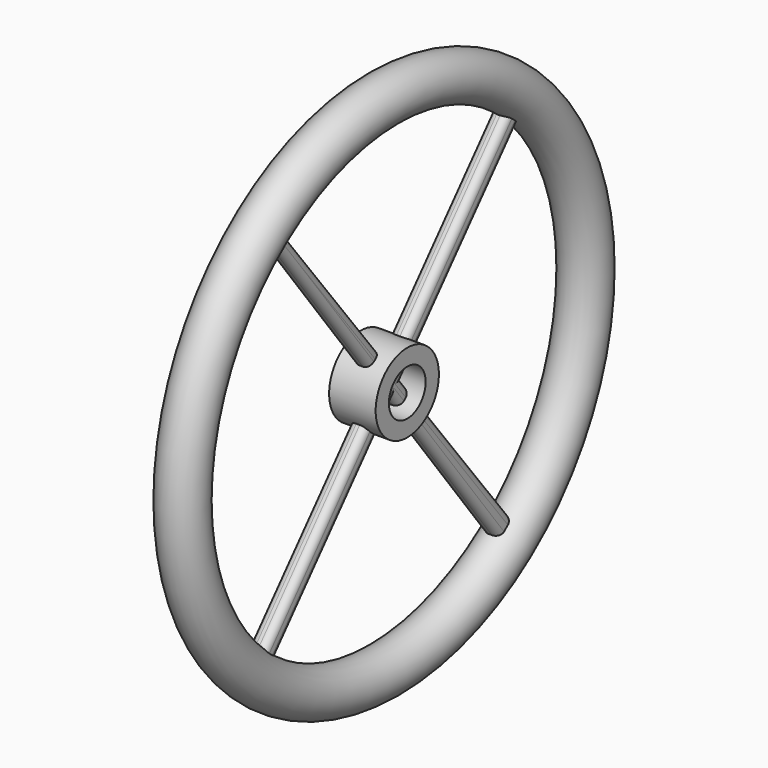
from build123d import *

# Parameters (mm, degrees)
F0_R          = 12.9236149617
F2_R          = 22.4555879502
F2_R_2        = 13.0373561963
F3_DEPTH      = 13.208
F5_DEPTH      = 4.826
F6_T1_DEPTH   = 9.652
F6_T3_DEPTH   = 28.9681227125
F6_T8_DEPTH   = 155.9510873217
F6_T13_DEPTH  = 155.9510873217
F6_T18_DEPTH  = 155.8155104326
F6_T23_DEPTH  = 155.8155104326
F6_T28_DEPTH  = 159.2863039853
F6_T33_DEPTH  = 159.2863039853
F6_T38_DEPTH  = 159.2863039853
F6_T43_DEPTH  = 159.2863039853
F6_T48_DEPTH  = 160.7409827394
F6_T53_DEPTH  = 160.7409827394
F6_T58_DEPTH  = 160.7409827394
F6_T63_DEPTH  = 160.7409827394
F6_T68_DEPTH  = 154.8184838298
F6_T73_DEPTH  = 154.8184838298
F6_T78_DEPTH  = 152.8193500484
F6_T83_DEPTH  = 152.8193500484
F6_T89_DEPTH  = 155.8155104326
F6_T93_DEPTH  = 155.9510873217
F6_T100_DEPTH = 155.8155104326
F6_T104_DEPTH = 155.9510873217
F6_T111_DEPTH = 154.8184838298
F6_T115_DEPTH = 159.2863039853
F6_T123_DEPTH = 154.8184838298
F6_T127_DEPTH = 159.2863039853
F6_T135_DEPTH = 151.0829213832
F6_T140_DEPTH = 143.1612886921
F6_T147_DEPTH = 151.0829213832
F6_T152_DEPTH = 143.1612886921
F6_T155_DEPTH = 144.3300677498
F6_T157_DEPTH = 146.2849391686
F6_T160_ANGLE = 78.1252953606
F6_T162_ANGLE = 78.1252953606


# Not quite as in the source:
# - a fillet or chamfer that OpenCascade refuses, or shapes differently, is made with other operations: its cross-section is extruded or revolved along the edge and cut away or added


with BuildPart() as f1:
    # F0 (on Front) → F1 (revolve)
    with BuildSketch(Plane.XZ):
        with Locations((0, 143.0430114269)):
            Circle(F0_R)
    revolve(axis=Axis((2.834841609, 0, 0), (1, 0, 0)))


with BuildPart() as f3:
    # F2 (on Right) → F3 (new body, symmetric)
    with BuildSketch(Plane.YZ):
        Circle(F2_R)
        Circle(F2_R_2, mode=Mode.SUBTRACT)
    extrude(amount=F3_DEPTH, both=True)


with BuildPart() as f5:
    # F4 (on Right) → F5 (new body, symmetric)
    with BuildSketch(Plane.YZ):
        Polygon((-83.4880173206, 116.8475523591), (-88.8398140669, 111.8525341153), (-5.84884804, 1.8371956864), (0.3858627438, 8.9852058397), align=None)
        Polygon((0.3858627438, 8.9852058397), (-5.84884804, 1.8371956864), (0.591610338, -6.7004710261), (6.9312324452, 0.5678185163), align=None)
        Polygon((0.591610338, -6.7004710261), (-5.84884804, 1.8371956864), (-100.2569794655, -106.4004283804), (-92.3700059439, -113.2796853781), align=None)
        Polygon((6.9312324452, 0.5678185163), (0.591610338, -6.7004710261), (80.9905081987, -113.2796853781), (90.1098596531, -106.4004283804), align=None)
        Polygon((90.1098596531, 111.8525341153), (0.3858627438, 8.9852058397), (6.9312324452, 0.5678185163), (98.9366569506, 106.0507721491), align=None)
    extrude(amount=F5_DEPTH, both=True)

    # F6: fillet of radius 3.8632245425 on 18 edges, made by hand

    # F6_s2 → F6_t1 (join)
    with BuildSketch(Plane.YZ.offset(-4.826)):
        with BuildLine():
            ThreePointArc((-7.9097995988, -0.5256569268), (-6.9603727243, 1.8766572944), (-7.7370489668, 4.3402520301))
            Line((-7.7370489668, 4.3402520301), (-5.84884804, 1.8371956864))
            Line((-5.84884804, 1.8371956864), (-7.9097995988, -0.5256569268))
        make_face()
    extrude(amount=F6_T1_DEPTH)

    # F6_s4 → F6_t3 (cut)
    with BuildSketch(Plane.YZ.offset(-14.4840613563)):
        with BuildLine():
            ThreePointArc((-97.7175985005, -103.489063034), (-98.6604928334, -106.2914766776), (-97.3456141191, -108.9398093454))
            Line((-97.3456141191, -108.9398093454), (-100.2569794655, -106.4004283804))
            Line((-100.2569794655, -106.4004283804), (-97.7175985005, -103.489063034))
        make_face()
    extrude(amount=F6_T3_DEPTH, mode=Mode.SUBTRACT)


with BuildPart() as f6_tool6:
    # F6_s7 → F6_t8 (new body)
    with BuildSketch(Plane(origin=(0, 1.7199108153, -2.2118163152), x_dir=(1, 0, 0), z_dir=(0, -0.6138537109, 0.7894198006))):
        with BuildLine():
            ThreePointArc((4.826, 1.9569850957), (3.6944877287, 4.688697367), (0.9627754575, 5.8202096382))
            Line((0.9627754575, 5.8202096382), (4.826, 5.8202096382))
            Line((4.826, 5.8202096382), (4.826, 1.9569850957))
        make_face()
    extrude(amount=F6_T8_DEPTH)

    split(bisect_by=Plane(origin=(0, -4.2318074253, 3.6911105082), x_dir=(1, 0, 0), z_dir=(0, -0.7536101809, 0.6573216071)), keep=Keep.TOP)


with BuildPart() as f5_1:
    add(f5.part)

    # F6_t5: cut F6_tool6
    add(f6_tool6.part, mode=Mode.SUBTRACT)


with BuildPart() as f6_tool11:
    # F6_s12 → F6_t13 (new body)
    with BuildSketch(Plane(origin=(0, 1.7199108153, -2.2118163152), x_dir=(1, 0, 0), z_dir=(0, -0.6138537109, 0.7894198006))):
        with BuildLine():
            ThreePointArc((-4.826, 1.9569850957), (-3.6944877287, 4.688697367), (-0.9627754575, 5.8202096382))
            Line((-0.9627754575, 5.8202096382), (-4.826, 5.8202096382))
            Line((-4.826, 5.8202096382), (-4.826, 1.9569850957))
        make_face()
    extrude(amount=F6_T13_DEPTH)

    split(bisect_by=Plane(origin=(0, -4.2318074253, 3.6911105082), x_dir=(1, 0, 0), z_dir=(0, -0.7536101809, 0.6573216071)), keep=Keep.TOP)


with BuildPart() as f5_2:
    add(f5_1.part)

    # F6_t10: cut F6_tool11
    add(f6_tool11.part, mode=Mode.SUBTRACT)


with BuildPart() as f6_tool16:
    # F6_s17 → F6_t18 (new body)
    with BuildSketch(Plane(origin=(0, 100.690119491, 115.4398369732), x_dir=(1, 0, 0), z_dir=(0, -0.6573216071, -0.7536101809))):
        with BuildLine():
            ThreePointArc((4.826, 1.7521553083), (3.6944877287, 4.4838675795), (0.9627754575, 5.6153798508))
            Line((0.9627754575, 5.6153798508), (4.826, 5.6153798508))
            Line((4.826, 5.6153798508), (4.826, 1.7521553083))
        make_face()
    extrude(amount=F6_T18_DEPTH)

    split(bisect_by=Plane(origin=(0, 4.5945887322, 3.5727572847), x_dir=(1, 0, 0), z_dir=(0, 0.7894198006, 0.6138537109)), keep=Keep.TOP)


with BuildPart() as f5_3:
    add(f5_2.part)

    # F6_t15: cut F6_tool16
    add(f6_tool16.part, mode=Mode.SUBTRACT)


with BuildPart() as f6_tool21:
    # F6_s22 → F6_t23 (new body)
    with BuildSketch(Plane(origin=(0, 100.690119491, 115.4398369732), x_dir=(1, 0, 0), z_dir=(0, -0.6573216071, -0.7536101809))):
        with BuildLine():
            ThreePointArc((-4.826, 1.7521553083), (-3.6944877287, 4.4838675795), (-0.9627754575, 5.6153798508))
            Line((-0.9627754575, 5.6153798508), (-4.826, 5.6153798508))
            Line((-4.826, 5.6153798508), (-4.826, 1.7521553083))
        make_face()
    extrude(amount=F6_T23_DEPTH)

    split(bisect_by=Plane(origin=(0, 4.5945887322, 3.5727572847), x_dir=(1, 0, 0), z_dir=(0, 0.7894198006, 0.6138537109)), keep=Keep.TOP)


with BuildPart() as f5_4:
    add(f5_3.part)

    # F6_t20: cut F6_tool21
    add(f6_tool21.part, mode=Mode.SUBTRACT)


with BuildPart() as f6_tool26:
    # F6_s27 → F6_t28 (new body)
    with BuildSketch(Plane(origin=(0, -3.0723860636, -3.5224483603), x_dir=(1, 0, 0), z_dir=(0, 0.6573216071, 0.7536101809))):
        with BuildLine():
            ThreePointArc((4.826, 0.9869834148), (3.6944877287, 3.7186956861), (0.9627754575, 4.8502079574))
            Line((0.9627754575, 4.8502079574), (4.826, 4.8502079574))
            Line((4.826, 4.8502079574), (4.826, 0.9869834148))
        make_face()
    extrude(amount=F6_T28_DEPTH)

    split(bisect_by=Plane(origin=(0, -2.8443496873, -2.1456583385), x_dir=(1, 0, 0), z_dir=(0, -0.7983268755, -0.6022243766)), keep=Keep.TOP)


with BuildPart() as f5_5:
    add(f5_4.part)

    # F6_t25: cut F6_tool26
    add(f6_tool26.part, mode=Mode.SUBTRACT)


with BuildPart() as f6_tool31:
    # F6_s32 → F6_t33 (new body)
    with BuildSketch(Plane(origin=(0, -3.0723860636, -3.5224483603), x_dir=(1, 0, 0), z_dir=(0, 0.6573216071, 0.7536101809))):
        with BuildLine():
            ThreePointArc((4.826, 0.9869834148), (3.6944877287, 3.7186956861), (0.9627754575, 4.8502079574))
            Line((0.9627754575, 4.8502079574), (4.826, 4.8502079574))
            Line((4.826, 4.8502079574), (4.826, 0.9869834148))
        make_face()
    extrude(amount=F6_T33_DEPTH)

    split(bisect_by=Plane(origin=(0, 4.5945887322, 3.5727572847), x_dir=(1, 0, 0), z_dir=(0, 0.7894198006, 0.6138537109)), keep=Keep.TOP)


with BuildPart() as f5_6:
    add(f5_5.part)

    # F6_t30: cut F6_tool31
    add(f6_tool31.part, mode=Mode.SUBTRACT)


with BuildPart() as f6_tool36:
    # F6_s37 → F6_t38 (new body)
    with BuildSketch(Plane(origin=(0, -3.0723860636, -3.5224483603), x_dir=(1, 0, 0), z_dir=(0, 0.6573216071, 0.7536101809))):
        with BuildLine():
            ThreePointArc((-4.826, 0.9869834148), (-3.6944877287, 3.7186956861), (-0.9627754575, 4.8502079574))
            Line((-0.9627754575, 4.8502079574), (-4.826, 4.8502079574))
            Line((-4.826, 4.8502079574), (-4.826, 0.9869834148))
        make_face()
    extrude(amount=F6_T38_DEPTH)

    split(bisect_by=Plane(origin=(0, -2.8443496873, -2.1456583385), x_dir=(1, 0, 0), z_dir=(0, -0.7983268755, -0.6022243766)), keep=Keep.TOP)


with BuildPart() as f5_7:
    add(f5_6.part)

    # F6_t35: cut F6_tool36
    add(f6_tool36.part, mode=Mode.SUBTRACT)


with BuildPart() as f6_tool41:
    # F6_s42 → F6_t43 (new body)
    with BuildSketch(Plane(origin=(0, -3.0723860636, -3.5224483603), x_dir=(1, 0, 0), z_dir=(0, 0.6573216071, 0.7536101809))):
        with BuildLine():
            ThreePointArc((-4.826, 0.9869834148), (-3.6944877287, 3.7186956861), (-0.9627754575, 4.8502079574))
            Line((-0.9627754575, 4.8502079574), (-4.826, 4.8502079574))
            Line((-4.826, 4.8502079574), (-4.826, 0.9869834148))
        make_face()
    extrude(amount=F6_T43_DEPTH)

    split(bisect_by=Plane(origin=(0, 4.5945887322, 3.5727572847), x_dir=(1, 0, 0), z_dir=(0, 0.7894198006, 0.6138537109)), keep=Keep.TOP)


with BuildPart() as f5_8:
    add(f5_7.part)

    # F6_t40: cut F6_tool41
    add(f6_tool41.part, mode=Mode.SUBTRACT)


with BuildPart() as f6_tool46:
    # F6_s47 → F6_t48 (new body)
    with BuildSketch(Plane(origin=(0, -102.3736244527, -117.3699522547), x_dir=(1, 0, 0), z_dir=(0, 0.6573216071, 0.7536101809))):
        with BuildLine():
            ThreePointArc((-4.826, 0.9869834148), (-3.6944877287, 3.7186956861), (-0.9627754575, 4.8502079574))
            Line((-0.9627754575, 4.8502079574), (-4.826, 4.8502079574))
            Line((-4.826, 4.8502079574), (-4.826, 0.9869834148))
        make_face()
    extrude(amount=F6_T48_DEPTH)

    split(bisect_by=Plane(origin=(0, -2.8443496873, -2.1456583385), x_dir=(1, 0, 0), z_dir=(0, -0.7983268755, -0.6022243766)), keep=Keep.TOP)


with BuildPart() as f5_9:
    add(f5_8.part)

    # F6_t45: cut F6_tool46
    add(f6_tool46.part, mode=Mode.SUBTRACT)


with BuildPart() as f6_tool51:
    # F6_s52 → F6_t53 (new body)
    with BuildSketch(Plane(origin=(0, -102.3736244527, -117.3699522547), x_dir=(1, 0, 0), z_dir=(0, 0.6573216071, 0.7536101809))):
        with BuildLine():
            ThreePointArc((-4.826, 0.9869834148), (-3.6944877287, 3.7186956861), (-0.9627754575, 4.8502079574))
            Line((-0.9627754575, 4.8502079574), (-4.826, 4.8502079574))
            Line((-4.826, 4.8502079574), (-4.826, 0.9869834148))
        make_face()
    extrude(amount=F6_T53_DEPTH)

    split(bisect_by=Plane(origin=(0, 4.5945887322, 3.5727572847), x_dir=(1, 0, 0), z_dir=(0, 0.7894198006, 0.6138537109)), keep=Keep.TOP)


with BuildPart() as f5_10:
    add(f5_9.part)

    # F6_t50: cut F6_tool51
    add(f6_tool51.part, mode=Mode.SUBTRACT)


with BuildPart() as f6_tool56:
    # F6_s57 → F6_t58 (new body)
    with BuildSketch(Plane(origin=(0, -102.3736244527, -117.3699522547), x_dir=(1, 0, 0), z_dir=(0, 0.6573216071, 0.7536101809))):
        with BuildLine():
            ThreePointArc((4.826, 0.9869834148), (3.6944877287, 3.7186956861), (0.9627754575, 4.8502079574))
            Line((0.9627754575, 4.8502079574), (4.826, 4.8502079574))
            Line((4.826, 4.8502079574), (4.826, 0.9869834148))
        make_face()
    extrude(amount=F6_T58_DEPTH)

    split(bisect_by=Plane(origin=(0, -2.8443496873, -2.1456583385), x_dir=(1, 0, 0), z_dir=(0, -0.7983268755, -0.6022243766)), keep=Keep.TOP)


with BuildPart() as f5_11:
    add(f5_10.part)

    # F6_t55: cut F6_tool56
    add(f6_tool56.part, mode=Mode.SUBTRACT)


with BuildPart() as f6_tool61:
    # F6_s62 → F6_t63 (new body)
    with BuildSketch(Plane(origin=(0, -102.3736244527, -117.3699522547), x_dir=(1, 0, 0), z_dir=(0, 0.6573216071, 0.7536101809))):
        with BuildLine():
            ThreePointArc((4.826, 0.9869834148), (3.6944877287, 3.7186956861), (0.9627754575, 4.8502079574))
            Line((0.9627754575, 4.8502079574), (4.826, 4.8502079574))
            Line((4.826, 4.8502079574), (4.826, 0.9869834148))
        make_face()
    extrude(amount=F6_T63_DEPTH)

    split(bisect_by=Plane(origin=(0, 4.5945887322, 3.5727572847), x_dir=(1, 0, 0), z_dir=(0, 0.7894198006, 0.6138537109)), keep=Keep.TOP)


with BuildPart() as f5_12:
    add(f5_11.part)

    # F6_t60: cut F6_tool61
    add(f6_tool61.part, mode=Mode.SUBTRACT)


with BuildPart() as f6_tool66:
    # F6_s67 → F6_t68 (new body)
    with BuildSketch(Plane(origin=(0, 91.4439077246, -117.5974505353), x_dir=(1, 0, 0), z_dir=(0, -0.6138537109, 0.7894198006))):
        with BuildLine():
            ThreePointArc((-4.826, 1.9569850957), (-3.6944877287, 4.688697367), (-0.9627754575, 5.8202096382))
            Line((-0.9627754575, 5.8202096382), (-4.826, 5.8202096382))
            Line((-4.826, 5.8202096382), (-4.826, 1.9569850957))
        make_face()
    extrude(amount=F6_T68_DEPTH)

    split(bisect_by=Plane(origin=(0, 3.6551660963, -3.1881464895), x_dir=(1, 0, 0), z_dir=(0, 0.7536101809, -0.6573216071)), keep=Keep.TOP)


with BuildPart() as f5_13:
    add(f5_12.part)

    # F6_t65: cut F6_tool66
    add(f6_tool66.part, mode=Mode.SUBTRACT)


with BuildPart() as f6_tool71:
    # F6_s72 → F6_t73 (new body)
    with BuildSketch(Plane(origin=(0, 91.4439077246, -117.5974505353), x_dir=(1, 0, 0), z_dir=(0, -0.6138537109, 0.7894198006))):
        with BuildLine():
            ThreePointArc((4.826, 1.9569850957), (3.6944877287, 4.688697367), (0.9627754575, 5.8202096382))
            Line((0.9627754575, 5.8202096382), (4.826, 5.8202096382))
            Line((4.826, 5.8202096382), (4.826, 1.9569850957))
        make_face()
    extrude(amount=F6_T73_DEPTH)

    split(bisect_by=Plane(origin=(0, 3.6551660963, -3.1881464895), x_dir=(1, 0, 0), z_dir=(0, 0.7536101809, -0.6573216071)), keep=Keep.TOP)


with BuildPart() as f5_14:
    add(f5_13.part)

    # F6_t70: cut F6_tool71
    add(f6_tool71.part, mode=Mode.SUBTRACT)


with BuildPart() as f6_tool76:
    # F6_s77 → F6_t78 (new body)
    with BuildSketch(Plane(origin=(0, -2.3803599544, 3.1554772586), x_dir=(1, 0, 0), z_dir=(0, 0.6022243766, -0.7983268755))):
        with BuildLine():
            ThreePointArc((-4.826, -0.3003359883), (-3.6944877287, 2.4313762829), (-0.9627754575, 3.5628885542))
            Line((-0.9627754575, 3.5628885542), (-4.826, 3.5628885542))
            Line((-4.826, 3.5628885542), (-4.826, -0.3003359883))
        make_face()
    extrude(amount=F6_T78_DEPTH)

    split(bisect_by=Plane(origin=(0, 3.6551660963, -3.1881464895), x_dir=(1, 0, 0), z_dir=(0, 0.7536101809, -0.6573216071)), keep=Keep.TOP)


with BuildPart() as f5_15:
    add(f5_14.part)

    # F6_t75: cut F6_tool76
    add(f6_tool76.part, mode=Mode.SUBTRACT)


with BuildPart() as f6_tool81:
    # F6_s82 → F6_t83 (new body)
    with BuildSketch(Plane(origin=(0, -2.3803599544, 3.1554772586), x_dir=(1, 0, 0), z_dir=(0, 0.6022243766, -0.7983268755))):
        with BuildLine():
            ThreePointArc((4.826, -0.3003359883), (3.6944877287, 2.4313762829), (0.9627754575, 3.5628885542))
            Line((0.9627754575, 3.5628885542), (4.826, 3.5628885542))
            Line((4.826, 3.5628885542), (4.826, -0.3003359883))
        make_face()
    extrude(amount=F6_T83_DEPTH)

    split(bisect_by=Plane(origin=(0, 3.6551660963, -3.1881464895), x_dir=(1, 0, 0), z_dir=(0, 0.7536101809, -0.6573216071)), keep=Keep.TOP)


with BuildPart() as f5_16:
    add(f5_15.part)

    # F6_t80: cut F6_tool81
    add(f6_tool81.part, mode=Mode.SUBTRACT)


with BuildPart() as f6_tool87:
    # F6_s88 → F6_t89 (new body)
    with BuildSketch(Plane(origin=(0, 100.690119491, 115.4398369732), x_dir=(1, 0, 0), z_dir=(0, -0.6573216071, -0.7536101809))):
        with BuildLine():
            ThreePointArc((4.826, 1.7521553083), (3.6944877287, 4.4838675795), (0.9627754575, 5.6153798508))
            Line((0.9627754575, 5.6153798508), (4.826, 5.6153798508))
            Line((4.826, 5.6153798508), (4.826, 1.7521553083))
        make_face()
    extrude(amount=F6_T89_DEPTH)

    split(bisect_by=Plane(origin=(0, 4.5945887322, 3.5727572847), x_dir=(1, 0, 0), z_dir=(0, -0.7894198006, -0.6138537109)), keep=Keep.TOP)


with BuildPart() as f6_tool91:
    # F6_s92 → F6_t93 (new body)
    with BuildSketch(Plane(origin=(0, 1.7199108153, -2.2118163152), x_dir=(1, 0, 0), z_dir=(0, -0.6138537109, 0.7894198006))):
        with BuildLine():
            ThreePointArc((4.826, 1.9569850957), (3.6944877287, 4.688697367), (0.9627754575, 5.8202096382))
            Line((0.9627754575, 5.8202096382), (4.826, 5.8202096382))
            Line((4.826, 5.8202096382), (4.826, 1.9569850957))
        make_face()
    extrude(amount=F6_T93_DEPTH)

    split(bisect_by=Plane(origin=(0, -4.2318074253, 3.6911105082), x_dir=(1, 0, 0), z_dir=(0, 0.7536101809, -0.6573216071)), keep=Keep.TOP)


with BuildPart() as f6_tool87_1:
    add(f6_tool87.part)

    # F6_t95: intersect F6_tool91
    add(f6_tool91.part, mode=Mode.INTERSECT)


with BuildPart() as f5_17:
    add(f5_16.part)

    # F6_t85: cut F6_tool87
    add(f6_tool87_1.part, mode=Mode.SUBTRACT)


with BuildPart() as f6_tool98:
    # F6_s99 → F6_t100 (new body)
    with BuildSketch(Plane(origin=(0, 100.690119491, 115.4398369732), x_dir=(1, 0, 0), z_dir=(0, -0.6573216071, -0.7536101809))):
        with BuildLine():
            ThreePointArc((-4.826, 1.7521553083), (-3.6944877287, 4.4838675795), (-0.9627754575, 5.6153798508))
            Line((-0.9627754575, 5.6153798508), (-4.826, 5.6153798508))
            Line((-4.826, 5.6153798508), (-4.826, 1.7521553083))
        make_face()
    extrude(amount=F6_T100_DEPTH)

    split(bisect_by=Plane(origin=(0, 4.5945887322, 3.5727572847), x_dir=(1, 0, 0), z_dir=(0, -0.7894198006, -0.6138537109)), keep=Keep.TOP)


with BuildPart() as f6_tool102:
    # F6_s103 → F6_t104 (new body)
    with BuildSketch(Plane(origin=(0, 1.7199108153, -2.2118163152), x_dir=(1, 0, 0), z_dir=(0, -0.6138537109, 0.7894198006))):
        with BuildLine():
            ThreePointArc((-4.826, 1.9569850957), (-3.6944877287, 4.688697367), (-0.9627754575, 5.8202096382))
            Line((-0.9627754575, 5.8202096382), (-4.826, 5.8202096382))
            Line((-4.826, 5.8202096382), (-4.826, 1.9569850957))
        make_face()
    extrude(amount=F6_T104_DEPTH)

    split(bisect_by=Plane(origin=(0, -4.2318074253, 3.6911105082), x_dir=(1, 0, 0), z_dir=(0, 0.7536101809, -0.6573216071)), keep=Keep.TOP)


with BuildPart() as f6_tool98_1:
    add(f6_tool98.part)

    # F6_t106: intersect F6_tool102
    add(f6_tool102.part, mode=Mode.INTERSECT)


with BuildPart() as f5_18:
    add(f5_17.part)

    # F6_t96: cut F6_tool98
    add(f6_tool98_1.part, mode=Mode.SUBTRACT)


with BuildPart() as f6_tool109:
    # F6_s110 → F6_t111 (new body)
    with BuildSketch(Plane(origin=(0, 91.4439077246, -117.5974505353), x_dir=(1, 0, 0), z_dir=(0, -0.6138537109, 0.7894198006))):
        with BuildLine():
            ThreePointArc((4.826, 1.9569850957), (3.6944877287, 4.688697367), (0.9627754575, 5.8202096382))
            Line((0.9627754575, 5.8202096382), (4.826, 5.8202096382))
            Line((4.826, 5.8202096382), (4.826, 1.9569850957))
        make_face()
    extrude(amount=F6_T111_DEPTH)

    split(bisect_by=Plane(origin=(0, 3.6551660963, -3.1881464895), x_dir=(1, 0, 0), z_dir=(0, -0.7536101809, 0.6573216071)), keep=Keep.TOP)


with BuildPart() as f6_tool113:
    # F6_s114 → F6_t115 (new body)
    with BuildSketch(Plane(origin=(0, -3.0723860636, -3.5224483603), x_dir=(1, 0, 0), z_dir=(0, 0.6573216071, 0.7536101809))):
        with BuildLine():
            ThreePointArc((4.826, 0.9869834148), (3.6944877287, 3.7186956861), (0.9627754575, 4.8502079574))
            Line((0.9627754575, 4.8502079574), (4.826, 4.8502079574))
            Line((4.826, 4.8502079574), (4.826, 0.9869834148))
        make_face()
    extrude(amount=F6_T115_DEPTH)

    split(bisect_by=Plane(origin=(0, -2.8443496873, -2.1456583385), x_dir=(1, 0, 0), z_dir=(0, 0.7983268755, 0.6022243766)), keep=Keep.TOP)

    split(bisect_by=Plane(origin=(0, 4.5945887322, 3.5727572847), x_dir=(1, 0, 0), z_dir=(0, -0.7894198006, -0.6138537109)), keep=Keep.TOP)


with BuildPart() as f6_tool109_1:
    add(f6_tool109.part)

    # F6_t118: intersect F6_tool113
    add(f6_tool113.part, mode=Mode.INTERSECT)


with BuildPart() as f5_19:
    add(f5_18.part)

    # F6_t107: cut F6_tool109
    add(f6_tool109_1.part, mode=Mode.SUBTRACT)


with BuildPart() as f6_tool121:
    # F6_s122 → F6_t123 (new body)
    with BuildSketch(Plane(origin=(0, 91.4439077246, -117.5974505353), x_dir=(1, 0, 0), z_dir=(0, -0.6138537109, 0.7894198006))):
        with BuildLine():
            ThreePointArc((-4.826, 1.9569850957), (-3.6944877287, 4.688697367), (-0.9627754575, 5.8202096382))
            Line((-0.9627754575, 5.8202096382), (-4.826, 5.8202096382))
            Line((-4.826, 5.8202096382), (-4.826, 1.9569850957))
        make_face()
    extrude(amount=F6_T123_DEPTH)

    split(bisect_by=Plane(origin=(0, 3.6551660963, -3.1881464895), x_dir=(1, 0, 0), z_dir=(0, -0.7536101809, 0.6573216071)), keep=Keep.TOP)


with BuildPart() as f6_tool125:
    # F6_s126 → F6_t127 (new body)
    with BuildSketch(Plane(origin=(0, -3.0723860636, -3.5224483603), x_dir=(1, 0, 0), z_dir=(0, 0.6573216071, 0.7536101809))):
        with BuildLine():
            ThreePointArc((-4.826, 0.9869834148), (-3.6944877287, 3.7186956861), (-0.9627754575, 4.8502079574))
            Line((-0.9627754575, 4.8502079574), (-4.826, 4.8502079574))
            Line((-4.826, 4.8502079574), (-4.826, 0.9869834148))
        make_face()
    extrude(amount=F6_T127_DEPTH)

    split(bisect_by=Plane(origin=(0, -2.8443496873, -2.1456583385), x_dir=(1, 0, 0), z_dir=(0, 0.7983268755, 0.6022243766)), keep=Keep.TOP)

    split(bisect_by=Plane(origin=(0, 4.5945887322, 3.5727572847), x_dir=(1, 0, 0), z_dir=(0, -0.7894198006, -0.6138537109)), keep=Keep.TOP)


with BuildPart() as f6_tool121_1:
    add(f6_tool121.part)

    # F6_t130: intersect F6_tool125
    add(f6_tool125.part, mode=Mode.INTERSECT)


with BuildPart() as f5_20:
    add(f5_19.part)

    # F6_t119: cut F6_tool121
    add(f6_tool121_1.part, mode=Mode.SUBTRACT)


with BuildPart() as f6_tool133:
    # F6_s134 → F6_t135 (new body)
    with BuildSketch(Plane(origin=(0, -96.0251720402, -110.0915388886), x_dir=(1, 0, 0), z_dir=(0, 0.6573216071, 0.7536101809))):
        with BuildLine():
            ThreePointArc((-4.826, 0.9869834148), (-3.6944877287, 3.7186956861), (-0.9627754575, 4.8502079574))
            Line((-0.9627754575, 4.8502079574), (-4.826, 4.8502079574))
            Line((-4.826, 4.8502079574), (-4.826, 0.9869834148))
        make_face()
    extrude(amount=F6_T135_DEPTH)

    split(bisect_by=Plane(origin=(0, -2.8443496873, -2.1456583385), x_dir=(1, 0, 0), z_dir=(0, 0.7983268755, 0.6022243766)), keep=Keep.TOP)

    split(bisect_by=Plane(origin=(0, 4.5945887322, 3.5727572847), x_dir=(1, 0, 0), z_dir=(0, -0.7894198006, -0.6138537109)), keep=Keep.TOP)


with BuildPart() as f6_tool138:
    # F6_s139 → F6_t140 (new body)
    with BuildSketch(Plane(origin=(0, -2.3803599544, 3.1554772586), x_dir=(1, 0, 0), z_dir=(0, 0.6022243766, -0.7983268755))):
        with BuildLine():
            ThreePointArc((-4.826, -0.3003359883), (-3.6944877287, 2.4313762829), (-0.9627754575, 3.5628885542))
            Line((-0.9627754575, 3.5628885542), (-4.826, 3.5628885542))
            Line((-4.826, 3.5628885542), (-4.826, -0.3003359883))
        make_face()
    extrude(amount=F6_T140_DEPTH)

    split(bisect_by=Plane(origin=(0, 3.6551660963, -3.1881464895), x_dir=(1, 0, 0), z_dir=(0, -0.7536101809, 0.6573216071)), keep=Keep.TOP)


with BuildPart() as f6_tool133_1:
    add(f6_tool133.part)

    # F6_t142: intersect F6_tool138
    add(f6_tool138.part, mode=Mode.INTERSECT)


with BuildPart() as f5_21:
    add(f5_20.part)

    # F6_t131: cut F6_tool133
    add(f6_tool133_1.part, mode=Mode.SUBTRACT)


with BuildPart() as f6_tool145:
    # F6_s146 → F6_t147 (new body)
    with BuildSketch(Plane(origin=(0, -96.0251720402, -110.0915388886), x_dir=(1, 0, 0), z_dir=(0, 0.6573216071, 0.7536101809))):
        with BuildLine():
            ThreePointArc((4.826, 0.9869834148), (3.6944877287, 3.7186956861), (0.9627754575, 4.8502079574))
            Line((0.9627754575, 4.8502079574), (4.826, 4.8502079574))
            Line((4.826, 4.8502079574), (4.826, 0.9869834148))
        make_face()
    extrude(amount=F6_T147_DEPTH)

    split(bisect_by=Plane(origin=(0, -2.8443496873, -2.1456583385), x_dir=(1, 0, 0), z_dir=(0, 0.7983268755, 0.6022243766)), keep=Keep.TOP)

    split(bisect_by=Plane(origin=(0, 4.5945887322, 3.5727572847), x_dir=(1, 0, 0), z_dir=(0, -0.7894198006, -0.6138537109)), keep=Keep.TOP)


with BuildPart() as f6_tool150:
    # F6_s151 → F6_t152 (new body)
    with BuildSketch(Plane(origin=(0, -2.3803599544, 3.1554772586), x_dir=(1, 0, 0), z_dir=(0, 0.6022243766, -0.7983268755))):
        with BuildLine():
            ThreePointArc((4.826, -0.3003359883), (3.6944877287, 2.4313762829), (0.9627754575, 3.5628885542))
            Line((0.9627754575, 3.5628885542), (4.826, 3.5628885542))
            Line((4.826, 3.5628885542), (4.826, -0.3003359883))
        make_face()
    extrude(amount=F6_T152_DEPTH)

    split(bisect_by=Plane(origin=(0, 3.6551660963, -3.1881464895), x_dir=(1, 0, 0), z_dir=(0, -0.7536101809, 0.6573216071)), keep=Keep.TOP)


with BuildPart() as f6_tool145_1:
    add(f6_tool145.part)

    # F6_t154: intersect F6_tool150
    add(f6_tool150.part, mode=Mode.INTERSECT)


with BuildPart() as f5_22:
    add(f5_21.part)

    # F6_t143: cut F6_tool145
    add(f6_tool145_1.part, mode=Mode.SUBTRACT)

    # F6_s156 → F6_t155 (cut)
    with BuildSketch(Plane(origin=(0, -91.8117843593, 121.7084824001), x_dir=(1, 0, 0), z_dir=(0, 0.6022243766, -0.7983268755))):
        with BuildLine():
            ThreePointArc((0.9627754575, 3.5628885542), (3.6944877287, 2.4313762829), (4.826, -0.3003359883))
            Line((4.826, -0.3003359883), (4.826, 3.5628885542))
            Line((4.826, 3.5628885542), (0.9627754575, 3.5628885542))
        make_face()
        with BuildLine():
            ThreePointArc((-4.826, -0.3003359883), (-3.6944877287, 2.4313762829), (-0.9627754575, 3.5628885542))
            Line((-0.9627754575, 3.5628885542), (-4.826, 3.5628885542))
            Line((-4.826, 3.5628885542), (-4.826, -0.3003359883))
        make_face()
    extrude(amount=F6_T155_DEPTH, mode=Mode.SUBTRACT)

    # F6_s158 → F6_t157 (cut)
    with BuildSketch(Plane(origin=(0, -3.6779921735, -4.216767435), x_dir=(1, 0, 0), z_dir=(0, -0.6573216071, -0.7536101809))):
        with BuildLine():
            ThreePointArc((-4.826, 1.7521553083), (-3.6944877287, 4.4838675795), (-0.9627754575, 5.6153798508))
            Line((-0.9627754575, 5.6153798508), (-4.826, 5.6153798508))
            Line((-4.826, 5.6153798508), (-4.826, 1.7521553083))
        make_face()
        with BuildLine():
            ThreePointArc((0.9627754575, 5.6153798508), (3.6944877287, 4.4838675795), (4.826, 1.7521553083))
            Line((4.826, 1.7521553083), (4.826, 5.6153798508))
            Line((4.826, 5.6153798508), (0.9627754575, 5.6153798508))
        make_face()
    extrude(amount=F6_T157_DEPTH, mode=Mode.SUBTRACT)

    # F6_s159 → F6_t160 (revolve, cut)
    with BuildSketch(Plane(origin=(0, -3.6779921735, -4.216767435), x_dir=(1, 0, 0), z_dir=(0, -0.6573216071, -0.7536101809))):
        with BuildLine():
            ThreePointArc((0.9627754575, 5.6153798508), (3.6944877287, 4.4838675795), (4.826, 1.7521553083))
            Line((4.826, 1.7521553083), (4.826, 5.6153798508))
            Line((4.826, 5.6153798508), (0.9627754575, 5.6153798508))
        make_face()
    revolve(axis=Axis((4.826, -10.8211649452, 2.0137240382), (1, 0, 0)), revolution_arc=F6_T160_ANGLE, mode=Mode.SUBTRACT)

    # F6_s161 → F6_t162 (revolve, cut)
    with BuildSketch(Plane(origin=(0, -3.6779921735, -4.216767435), x_dir=(1, 0, 0), z_dir=(0, -0.6573216071, -0.7536101809))):
        with BuildLine():
            ThreePointArc((-4.826, 1.7521553083), (-3.6944877287, 4.4838675795), (-0.9627754575, 5.6153798508))
            Line((-0.9627754575, 5.6153798508), (-4.826, 5.6153798508))
            Line((-4.826, 5.6153798508), (-4.826, 1.7521553083))
        make_face()
    revolve(axis=Axis((-4.826, -10.8211649452, 2.0137240382), (1, 0, 0)), revolution_arc=F6_T162_ANGLE, mode=Mode.SUBTRACT)


solid = Compound([f1.part, f3.part, f5_22.part])
